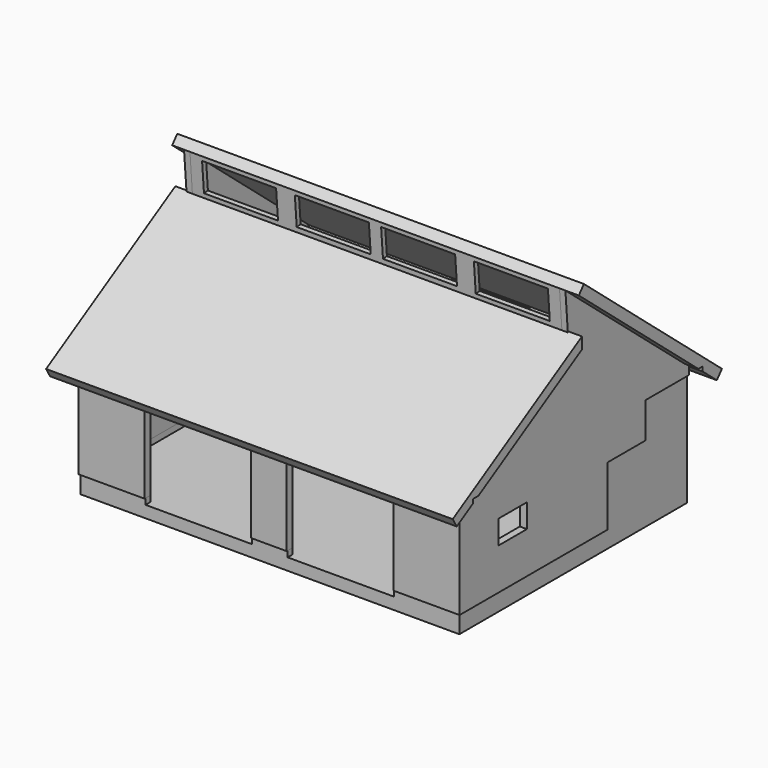
from build123d import *

# Parameters (mm, degrees)
F0_W           = 9753.6
F0_H           = 7315.2
F1_DEPTH       = 304.8
F2_W           = 914.4
F2_H           = 152.4
F3_DEPTH       = 152.4
F5_DEPTH       = 2438.4
F7_DEPTH       = 152.4
F9_DEPTH       = 152.4
F10_W          = 914.4
F10_H          = 609.6
F11_DEPTH      = 152.4
F11_DEPTH_BACK = 30.48
F13_DEPTH      = 152.4
F13_DEPTH_BACK = 30.48
F14_W          = 914.4
F14_H          = 609.6
F15_DEPTH      = 182.88
F16_W          = 9814.56
F16_H          = 7376.16
F16_W_2        = 2032
F16_H_2        = 914.4
F17_DEPTH      = 304.8
F19_DEPTH      = 914.4
F24_DEPTH      = 304.8
F24_DEPTH_BACK = 10160
F26_DEPTH      = 152.4
F28_DEPTH      = 152.4
F29_W          = 9814.56
F29_H          = 985.611441973
F29_W_2        = 1905
F29_H_2        = 762
F29_H_3        = 749.1830940247
F30_DEPTH      = 127


with BuildPart() as f1:
    # F0 (on Top) → F1 (new body)
    with BuildSketch(Plane.XY):
        with Locations((4876.8, 3657.6)):
            Rectangle(F0_W, F0_H)
    extrude(amount=F1_DEPTH)

    # F2 (on face) → F3 (join)
    with BuildSketch(Plane.XY.offset(304.8)):
        with Locations((4876.8, 76.2)):
            Rectangle(F2_W, F2_H)
        Polygon((8077.2, 152.4), (8077.2, 0), (9753.6, 0), (9753.6, 7315.2), (0, 7315.2), (0, 1371.6), (152.4, 1371.6), (152.4, 7162.8), (9601.2, 7162.8), (9601.2, 152.4), align=None)
        Polygon((0, 0), (1676.4, 0), (1676.4, 152.4), (152.4, 152.4), (152.4, 457.2), (0, 457.2), align=None)
    extrude(amount=F3_DEPTH)

    # F4 (on face) → F5 (join)
    with BuildSketch(Plane.XY.offset(457.2)):
        Polygon((0, 7315.2), (0, 7162.8), (9601.2, 7162.8), (9753.6, 7162.8), (9753.6, 7315.2), align=None)
    extrude(amount=F5_DEPTH)

    # F6 (on face) → F7 (join)
    with BuildSketch(Plane.YZ.offset(9753.6)):
        Polygon((4724.4, 1981.2), (4724.4, 457.2), (7162.8, 457.2), (7162.8, 2895.6), (5943.6, 2895.6), (5943.6, 1981.2), align=None)
    extrude(amount=-F7_DEPTH)

    # F8 (on face) → F9 (join)
    with BuildSketch(Plane(origin=(0, 0, 0), x_dir=(0, -1, 0), z_dir=(-1, 0, 0))):
        Polygon((-7162.8, 457.2), (-4114.8, 457.2), (-4114.8, 1676.4), (-5638.8, 1676.4), (-5638.8, 2895.6), (-7162.8, 2895.6), align=None)
    extrude(amount=-F9_DEPTH)


with BuildPart() as f11:
    # F10 (on face) → F11 (new body, two sides)
    with BuildSketch(Plane.YZ.offset(9753.6)) as f11_sk:
        Polygon((5943.6, 1981.2), (5943.6, 2895.6), (0, 2895.6), (0, 457.2), (4724.4, 457.2), (4724.4, 1981.2), align=None)
        with Locations((1676.4, 1828.8)):
            Rectangle(F10_W, F10_H, mode=Mode.SUBTRACT)
    extrude(amount=-F11_DEPTH)
    extrude(f11_sk.sketch, amount=F11_DEPTH_BACK)

    # F12 (on face) → F13 (join, two sides)
    with BuildSketch(Plane.XZ) as f13_sk:
        Polygon((-30.48, 457.2), (0, 457.2), (1676.4, 457.2), (1676.4, 2743.2), (4419.6, 2743.2), (4419.6, 457.2), (5334, 457.2), (5334, 2743.2), (8077.2, 2743.2), (8077.2, 457.2), (9601.2, 457.2), (9753.6, 457.2), (9784.08, 457.2), (9784.08, 2895.6), (9601.2, 2895.6), (152.4, 2895.6), (-30.48, 2895.6), align=None)
    extrude(amount=-F13_DEPTH)
    extrude(f13_sk.sketch, amount=F13_DEPTH_BACK)

    # F14 (on face) → F15 (join)
    with BuildSketch(Plane(origin=(-30.48, 0, 0), x_dir=(0, -1, 0), z_dir=(-1, 0, 0))):
        Polygon((30.48, 2895.6), (-5638.8, 2895.6), (-5638.8, 1676.4), (-4114.8, 1676.4), (-4114.8, 457.2), (-1371.6, 457.2), (-1371.6, 2438.4), (-457.2, 2438.4), (-457.2, 457.2), (30.48, 457.2), align=None)
        with Locations((-2865.12, 2133.6)):
            Rectangle(F14_W, F14_H, mode=Mode.SUBTRACT)
    extrude(amount=-F15_DEPTH)

    # F16 (on face) → F17 (join)
    with BuildSketch(Plane.XY.offset(2895.6)):
        with Locations((4876.8, 3657.6)):
            Rectangle(F16_W, F16_H)
        with Locations((4826, 6705.6)):
            Rectangle(F16_W_2, F16_H_2, mode=Mode.SUBTRACT)
    extrude(amount=F17_DEPTH)

    # F23 (on face) → F24 (join, two sides)
    with BuildSketch(Plane(origin=(-30.48, 0, 0), x_dir=(0, -1, 0), z_dir=(-1, 0, 0))) as f24_sk:
        Polygon((-7975.9287453857, 2895.6), (-7812.6606925253, 2701.0247114478), (-7345.68, 3092.8680383127), (-7345.68, 3200.4), (-7217.5283983405, 3200.4), (-3372.4119471396, 6426.8357960363), (-3535.68, 6621.4110845885), align=None)
        Polygon((684.6438803972, 3008.2584206913), (-3473.5784478936, 5457.6385603397), (-3473.5784478936, 5162.8481659781), (-142.0025729235, 3200.4), (30.48, 3200.4), (30.48, 3098.8), (555.7291362052, 2789.4046139392), align=None)
    extrude(amount=F24_DEPTH)
    extrude(f24_sk.sketch, amount=-F24_DEPTH_BACK)

    # F25 (on face) → F26 (join)
    with BuildSketch(Plane(origin=(-30.48, 0, 0), x_dir=(0, -1, 0), z_dir=(-1, 0, 0))):
        Polygon((-3372.4119471396, 6426.8357960363), (-7217.5283983405, 3200.4), (-142.0025729235, 3200.4), (-3473.5784478936, 5162.8481659781), align=None)
    extrude(amount=-F26_DEPTH)

    # F27 (on face) → F28 (join)
    with BuildSketch(Plane.YZ.offset(9784.08)):
        Polygon((142.0025729235, 3200.4), (7217.5283983404, 3200.4), (3372.4119471396, 6426.8357960363), (3473.5784478936, 5162.8481659781), align=None)
    extrude(amount=-F28_DEPTH)

    # F29 (on face) → F30 (join)
    with BuildSketch(Plane(origin=(0, 3862.0598735135, 309.1098946023), x_dir=(1, 0, 0), z_dir=(0, -0.9968123007, -0.0797824361))):
        with Locations((4876.8, 5644.4840144651)):
            Rectangle(F29_W, F29_H)
        with Locations((1379.22, 5647.3764953613)):
            Rectangle(F29_W_2, F29_H_2, mode=Mode.SUBTRACT)
        with Locations((3766.82, 5653.784948349)):
            Rectangle(F29_W_2, F29_H_3, mode=Mode.SUBTRACT)
        with Locations((5986.78, 5653.784948349)):
            Rectangle(F29_W_2, F29_H_3, mode=Mode.SUBTRACT)
        with Locations((8374.38, 5647.3764953613)):
            Rectangle(F29_W_2, F29_H_2, mode=Mode.SUBTRACT)
    extrude(amount=-F30_DEPTH)


with BuildPart() as f19:
    # F18 (on face) → F19 (new body)
    with BuildSketch(Plane.XZ.offset(-7162.8)):
        Polygon((1524, 482.6), (1524, 304.8), (2032, 304.8), (5943.6, 3149.6), (5435.6, 3149.6), (5435.6, 2959.1), (5156.2, 2959.1), (5156.2, 2768.6), (4876.8, 2768.6), (4876.8, 2578.1), (4597.4, 2578.1), (4597.4, 2387.6), (4318, 2387.6), (4318, 2197.1), (4038.6, 2197.1), (4038.6, 2006.6), (3759.2, 2006.6), (3759.2, 1816.1), (3479.8, 1816.1), (3479.8, 1625.6), (3200.4, 1625.6), (3200.4, 1435.1), (2921, 1435.1), (2921, 1244.6), (2641.6, 1244.6), (2641.6, 1054.1), (2362.2, 1054.1), (2362.2, 863.6), (2082.8, 863.6), (2082.8, 673.1), (1803.4, 673.1), (1803.4, 482.6), align=None)
    extrude(amount=F19_DEPTH)


solid = Compound([f1.part, f11.part, f19.part])
